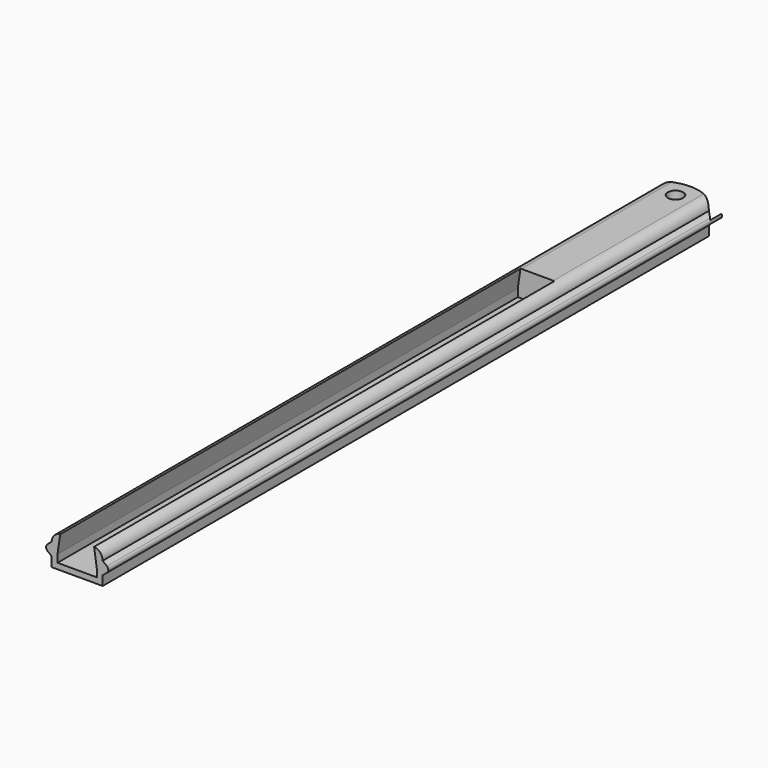
from build123d import *

# Parameters (mm, degrees)
F1_DEPTH = 200
F2_R     = 2
F3_DEPTH = 8.301
F6_DEPTH = 25
F9_DEPTH = 150


# Not quite as in the source:
# - a feature names something its author has since deleted; it is built from what else it names


with BuildPart() as f1:
    # F0 (on Front) → F1 (new body)
    with BuildSketch(Plane.XZ):
        with BuildLine():
            Line((7.7333916469, 0.7795584959), (6.65, 1.65))
            ThreePointArc((6.65, 1.65), (5.917766953, 3.417766953), (4.15, 4.15))
            Line((4.15, 4.15), (-4.15, 4.15))
            ThreePointArc((-4.15, 4.15), (-5.917766953, 3.417766953), (-6.65, 1.65))
            Line((-6.65, 1.65), (-7.7333916469, 0.7795584959))
            ThreePointArc((-7.7333916469, 0.7795584959), (-8.1070622196, 0), (-7.7333916469, -0.7795584959))
            Line((-7.7333916469, -0.7795584959), (-6.65, -1.65))
            Line((-6.65, -1.65), (-6.65, -4.15))
            Line((-6.65, -4.15), (-4.15, -4.15))
            Line((-4.15, -4.15), (4.15, -4.15))
            Line((4.15, -4.15), (6.65, -4.15))
            Line((6.65, -4.15), (6.65, -1.65))
            Line((6.65, -1.65), (7.7333916469, -0.7795584959))
            ThreePointArc((7.7333916469, -0.7795584959), (8.1070622196, 0), (7.7333916469, 0.7795584959))
        make_face()
        with BuildLine():
            ThreePointArc((5.15, -1.65), (4.8571067812, -2.3571067812), (4.15, -2.65))
            Line((4.15, -2.65), (-4.15, -2.65))
            ThreePointArc((-4.15, -2.65), (-4.8571067812, -2.3571067812), (-5.15, -1.65))
            Line((-5.15, -1.65), (-5.15, 1.65))
            ThreePointArc((-5.15, 1.65), (-4.8571067812, 2.3571067812), (-4.15, 2.65))
            Line((-4.15, 2.65), (4.15, 2.65))
            ThreePointArc((4.15, 2.65), (4.8571067812, 2.3571067812), (5.15, 1.65))
            Line((5.15, 1.65), (5.15, -1.65))
        make_face(mode=Mode.SUBTRACT)
        with BuildLine():
            Line((-4.15, -2.65), (4.15, -2.65))
            ThreePointArc((4.15, -2.65), (4.8571067812, -2.3571067812), (5.15, -1.65))
            Line((5.15, -1.65), (5.15, 1.65))
            ThreePointArc((5.15, 1.65), (4.8571067812, 2.3571067812), (4.15, 2.65))
            Line((4.15, 2.65), (-4.15, 2.65))
            ThreePointArc((-4.15, 2.65), (-4.8571067812, 2.3571067812), (-5.15, 1.65))
            Line((-5.15, 1.65), (-5.15, -1.65))
            ThreePointArc((-5.15, -1.65), (-4.8571067812, -2.3571067812), (-4.15, -2.65))
        make_face()
    extrude(amount=F1_DEPTH)

    # F2 (on face) → F3 (cut, through all)
    with BuildSketch(Plane.XY.offset(4.15)):
        with Locations((0, -5)):
            Circle(F2_R)
    extrude(amount=-F3_DEPTH, mode=Mode.SUBTRACT)

    # F5 (on offset) → F6 (cut)
    with BuildSketch(Plane.XY.offset(4.6)):
        with BuildLine():
            Line((8, -3.7011680724), (8, 3.7011680724))
            Line((8, 3.7011680724), (-8, 3.7011680724))
            Line((-8, 3.7011680724), (-8, -3.7011680724))
            ThreePointArc((-8, -3.7011680724), (0, -0.1482238292), (8, -3.7011680724))
        make_face()
    extrude(amount=-F6_DEPTH, mode=Mode.SUBTRACT)

    # F8 (on offset) → F9 (cut)
    with BuildSketch(Plane.XZ.offset(200)):
        Polygon((-5.1262229681, -2.646596171), (0, -2.646596171), (5.1262229681, -2.646596171), (5.1262229681, -0.6600963534), (4.3867812492, 4.353403829), (0, 4.353403829), (-4.3867812492, 4.353403829), (-5.1262229681, -0.6600963534), align=None)
    extrude(amount=-F9_DEPTH, mode=Mode.SUBTRACT)


solid = f1.part
